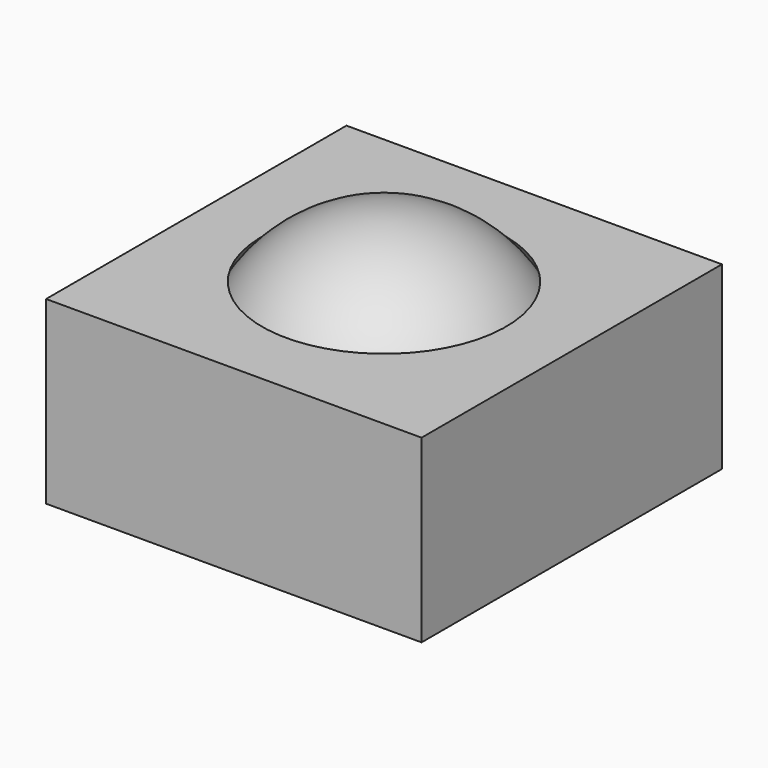
from build123d import *

# Parameters (mm, degrees)
F0_W     = 25
F0_H     = 25
F1_DEPTH = 12
F6_R     = 3.5
F7_DEPTH = 10


# Not quite as in the source:
# - a fillet or chamfer that OpenCascade refuses, or shapes differently, is made with other operations: its cross-section is extruded or revolved along the edge and cut away or added


with BuildPart() as f1:
    # F0 (on Top) → F1 (new body)
    with BuildSketch(Plane.XY):
        Rectangle(F0_W, F0_H)
    extrude(amount=F1_DEPTH)

    # F2 (on Right) → F3 (revolve, cut)
    with BuildSketch(Plane.YZ):
        with BuildLine():
            Line((0, 16.1), (0, -4.1))
            ThreePointArc((0, -4.1), (10.1, 6), (0, 16.1))
        make_face()
    revolve(axis=Axis((0, 0, 6), (0, 0, -1)), mode=Mode.SUBTRACT)

    # F8: chamfer of 0.2 on 1 edges, made by hand

    # F8_s1 → F8_t2 (revolve, cut)
    with BuildSketch(Plane.YZ):
        with BuildLine():
            Line((8.325924515, -0.0071067019), (8.2362376015, 0.1663991572))
            Line((8.2362376015, 0.1663991572), (8.2329742703, 0.1687123087))
            ThreePointArc((8.2329742703, 0.1687123087), (8.1804857118, 0.0831706532), (8.1214361541, 0.0023762376))
            Line((8.1214361541, 0.0023762376), (8.1246538388, -0.004))
            ThreePointArc((8.1246538388, -0.004), (8.2252891769, -0.004), (8.325924515, -0.0111067019))
            Line((8.325924515, -0.0111067019), (8.325924515, -0.0071067019))
        make_face()
    revolve(axis=Axis((0, 0, 0), (0, 0, 1)), mode=Mode.SUBTRACT)


with BuildPart() as f5:
    # F4 (on Right) → F5 (revolve)
    with BuildSketch(Plane.YZ):
        with BuildLine():
            Line((0, 0), (7.9374114168, 0))
            ThreePointArc((7.9374114168, 0), (8.9079318587, 10.432973043), (0, 15.95))
            Line((0, 15.95), (0, 0))
        make_face()
    revolve(axis=Axis((0, 0, 7.975), (0, 0, -1)))

    # F6 (on face) → F7 (cut)
    with BuildSketch(Plane(origin=(0, 0, 0), x_dir=(1, 0, 0), z_dir=(0, 0, -1))):
        Circle(F6_R)
    extrude(amount=-F7_DEPTH, mode=Mode.SUBTRACT)

    # F8#2: chamfer of 0.2 on 1 edges, made by hand

    # F8_2_s1 → F8_2_t2 (revolve, cut)
    with BuildSketch(Plane.YZ):
        with BuildLine():
            Line((7.7277014115, -0.0036384376), (8.0675214314, 0.169899927))
            Line((8.0675214314, 0.169899927), (8.0707617919, 0.1675547055))
            ThreePointArc((8.0707617919, 0.1675547055), (8.0046815514, 0.0833126447), (7.940602336, -0.0024120603))
            Line((7.940602336, -0.0024120603), (7.9374114168, -0.004))
            ThreePointArc((7.9374114168, -0.004), (7.8325564142, -0.004), (7.7277014115, -0.0076384376))
            Line((7.7277014115, -0.0076384376), (7.7277014115, -0.0036384376))
        make_face()
    revolve(axis=Axis((0, 0, 0), (0, 0, -1)), mode=Mode.SUBTRACT)


solid = Compound([f1.part, f5.part])
